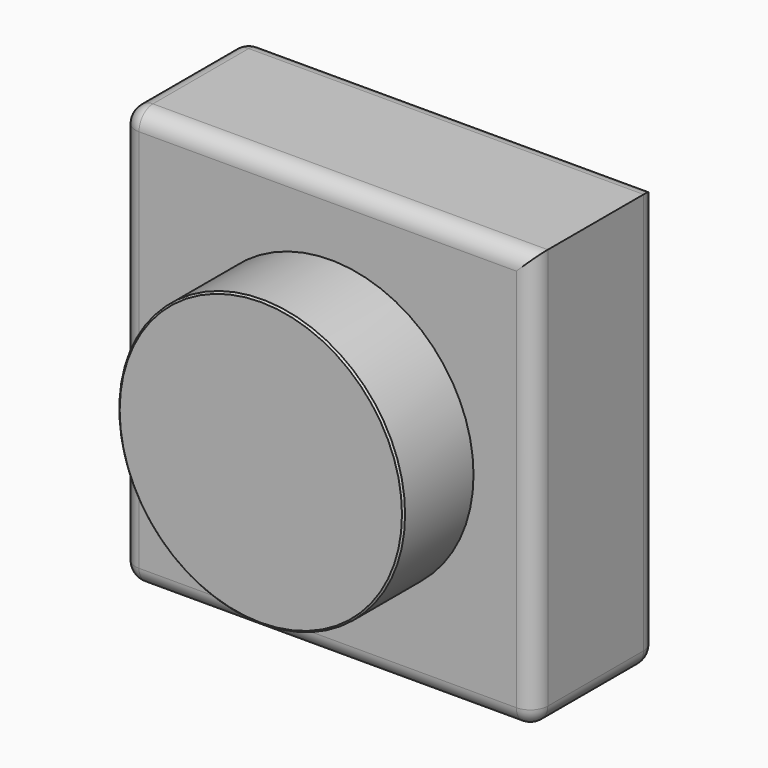
from build123d import *

# Parameters (mm, degrees)
F0_W      = 120
F0_H      = 121.996589005
F1_DEPTH  = 45
F3_R      = 35.3699694231
F2_R      = 41.5830123254
F4_DEPTH  = 50.8
F5_R      = 5.08
F6_DEPTH  = 25.4
F7_DEPTH  = 25.4
F9_DEPTH  = 25.4
F10_SIZE  = 0.5
F11_T     = 2.54
F12_R     = 35.1358269191
F13_DEPTH = 25.4


# Not quite as in the source:
# - a shell that OpenCascade refuses in one call is made with other operations: the cavity is built on its own and cut out
# - the program builds the solid bodies; features that only make, move or delete a surface that nothing else refers to are left out


with BuildPart() as f1:
    # F0 (on Front) → F1 (new body)
    with BuildSketch(Plane.XZ):
        with Locations((-0.8642734587, 0.3312714398)):
            Rectangle(F0_W, F0_H)
    extrude(amount=F1_DEPTH)

    # F3 (on face) + F2 (on face) → F4 (cut)
    with BuildSketch(Plane.XZ.offset(45)):
        Circle(F3_R)
    with BuildSketch(Plane.XZ.offset(45)):
        Circle(F2_R)
    extrude(amount=F4_DEPTH, mode=Mode.SUBTRACT)

    # F5
    f5_edges = [f1.edges().sort_by_distance(p)[0] for p in [
        (-60.864273, -22.5, 61.329566),
        (-60.864273, -22.5, -60.667023),
        (-60.864273, 0, 0.331271),
        (-60.864273, -45, 0.331271),
        (-0.864273, -45, 61.329566),
        (-0.864273, 0, 61.329566),
        (59.135727, 0, 0.331271),
        (59.135727, -45, 0.331271),
        (59.135727, -22.5, -60.667023),
        (-0.864273, -45, -60.667023),
        (-0.864273, 0, -60.667023),
    ]]
    fillet(f5_edges, radius=F5_R)

    # F3 (on face) + F2 (on face) → F6 (join)
    with BuildSketch(Plane.XZ.offset(45)):
        Circle(F3_R)
    with BuildSketch(Plane.XZ.offset(45)):
        Circle(F2_R)
    extrude(amount=F6_DEPTH)

    # F3 (on face) → F7 (join)
    with BuildSketch(Plane.XZ.offset(45)):
        Circle(F3_R)
    extrude(amount=-F7_DEPTH)

    # F3 (on face) → F9 (join)
    with BuildSketch(Plane.XZ.offset(45)):
        Circle(F3_R)
    extrude(amount=-F9_DEPTH)

    # F10
    f10_edges = [f1.edges().sort_by_distance(p)[0] for p in [
        (-41.583012, -70.4, 0),
    ]]
    chamfer(f10_edges, length=F10_SIZE)

    # F11: shell of thickness 2.54, made by hand


with BuildPart() as f11_core1:
    # F11_t2: copy of F1
    add(f1.part)

    # the walls: a layer under each face that stays
    f11_faces = [f11_core1.faces().sort_by_distance(p)[0] for p in [
        (-41.5830123254, -57.45, 0),
        (-41.3330123254, -70.15, 0),
        (-37.4776067921, -45, -36.9475915619),
        (0, -70.4, 0),
        (-59.3763759071, -43.5121024484, 0.3312714398),
        (1.6757265413, -43.5121025775, 59.8416682617),
        (-0.8642734587, -43.5121024484, -59.1791255111),
        (57.6478288607, -43.5121025775, 2.8712714398),
        (-58.3242734587, -43.5121024484, 58.7895659423),
        (-60.8642734587, -22.5, 0.3312714398),
        (-58.3242734587, -43.5121024484, -58.1270230627),
        (1.6757265413, -22.5, 61.3295659423),
        (-0.8642734587, -22.5, -60.6670230627),
        (56.5957265413, -42.46, -59.1791255111),
        (59.1357265413, -22.5, 2.8712714398),
        (-59.3763759071, -22.5, 59.8416683907),
        (-59.3763759071, -1.4878975516, 0.3312714398),
        (-59.3763759071, -22.5, -59.1791255111),
        (1.6757265413, -1.4878975516, 59.8416683907),
        (-0.8642734587, -1.4878975516, -59.1791255111),
        (57.6478289897, -22.5, -59.1791255111),
        (57.6478289897, -1.4878975516, 2.8712714398),
        (-58.3242734587, -1.4878975516, 58.7895659423),
        (-58.3242734587, -1.4878975516, -58.1270230627),
        (56.5957265413, -2.54, -59.1791255111),
    ]]
    thicken(f11_faces, amount=-F11_T, mode=Mode.SUBTRACT)

    # F11_s3 → F11_t4 (revolve, cut)
    with BuildSketch(Plane.XY):
        Polygon((41.6084123254, -45.0254), (39.0430123254, -45), (39.0430123254, -42.46), (41.5830123254, -42.46), align=None)
    revolve(axis=Axis((0, -45, 0), (0, -1, 0)), mode=Mode.SUBTRACT)


with BuildPart() as f1_1:
    add(f1.part)

    # what is left inside the walls is the cavity
    f11_cavity = [f11_core1.part.solids().sort_by_distance(p)[0] for p in [
        (-0.864273, -0.0254, -18.30816),
    ]]
    add(f11_cavity, mode=Mode.SUBTRACT)


with BuildPart() as f13:
    # F12 (on Front) → F13 (new body)
    with BuildSketch(Plane.XZ):
        Circle(F12_R)
    extrude(amount=F13_DEPTH)


solid = Compound([f1_1.part, f13.part])
